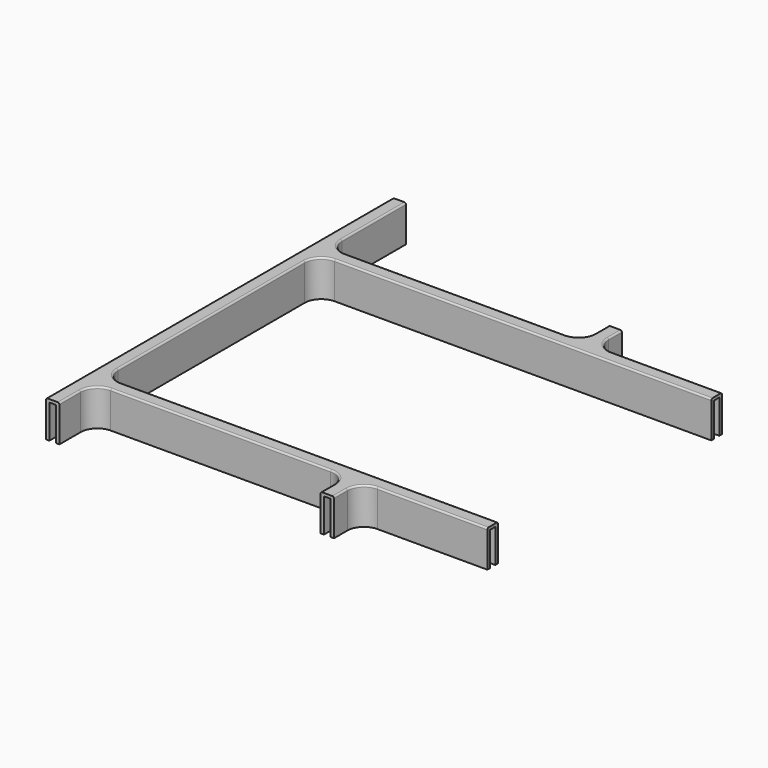
from build123d import *

# Parameters (mm, degrees)
F0_W     = 2
F0_H     = 10
F0_H_2   = 1
F1_DEPTH = 0.9
F0_W_2   = 1
F0_H_3   = 130
F0_W_3   = 76
F0_W_4   = 38
F2_DEPTH = 11
F3_R     = 5
F4_R     = 0.5


with BuildPart() as f1:
    # F0 (on Top) → F1 (new body)
    with BuildSketch(Plane.XY):
        Polygon((-1, -65), (1, -65), (1, -51), (1, -49), (1, 33), (1, 35), (1, 65), (-1, 65), align=None)
        Polygon((1, 35), (1, 33), (2, 33), (79, 33), (81, 33), (120, 33), (120, 35), (82, 35), (81, 35), (79, 35), (78, 35), (2, 35), align=None)
        with Locations((80, 41)):
            Rectangle(F0_W, F0_H)
        with Locations((80, 35.5)):
            Rectangle(F0_W, F0_H_2)
        Polygon((1, -49), (1, -51), (2, -51), (78, -51), (79, -51), (81, -51), (82, -51), (120, -51), (120, -49), (81, -49), (79, -49), (2, -49), align=None)
        with Locations((80, -57)):
            Rectangle(F0_W, F0_H)
        with Locations((80, -51.5)):
            Rectangle(F0_W, F0_H_2)
    extrude(amount=-F1_DEPTH)

    # F0 (on Top) → F2 (join)
    with BuildSketch(Plane.XY):
        Polygon((1, -51), (1, -65), (2, -65), (2, -52), (2, -51), align=None)
        with Locations((-1.5, 0)):
            Rectangle(F0_W_2, F0_H_3)
        Polygon((1, 33), (1, -49), (2, -49), (2, -48), (2, 32), (2, 33), align=None)
        with Locations((40, -51.5)):
            Rectangle(F0_W_3, F0_H_2)
        Polygon((2, 65), (1, 65), (1, 35), (2, 35), (2, 36), align=None)
        Polygon((2, -48), (2, -49), (79, -49), (79, -48), (78, -48), align=None)
        with Locations((78.5, -51.5)):
            Rectangle(F0_W_2, F0_H_2)
        with Locations((78.5, -57)):
            Rectangle(F0_W_2, F0_H)
        Polygon((79, 33), (2, 33), (2, 32), (78, 32), (79, 32), align=None)
        with Locations((80, -48.5)):
            Rectangle(F0_W, F0_H_2)
        with Locations((40, 35.5)):
            Rectangle(F0_W_3, F0_H_2)
        with Locations((80, 32.5)):
            Rectangle(F0_W, F0_H_2)
        Polygon((81, -48), (81, -49), (120, -49), (120, -48), (82, -48), align=None)
        with Locations((81.5, -51.5)):
            Rectangle(F0_W_2, F0_H_2)
        with Locations((81.5, -57)):
            Rectangle(F0_W_2, F0_H)
        with Locations((78.5, 35.5)):
            Rectangle(F0_W_2, F0_H_2)
        with Locations((78.5, 41)):
            Rectangle(F0_W_2, F0_H)
        Polygon((120, 33), (81, 33), (81, 32), (82, 32), (120, 32), align=None)
        with Locations((101, -51.5)):
            Rectangle(F0_W_4, F0_H_2)
        with Locations((81.5, 35.5)):
            Rectangle(F0_W_2, F0_H_2)
        with Locations((81.5, 41)):
            Rectangle(F0_W_2, F0_H)
        with Locations((101, 35.5)):
            Rectangle(F0_W_4, F0_H_2)
    extrude(amount=-F2_DEPTH)

    # F3
    f3_edges = [f1.edges().sort_by_distance(p)[0] for p in [
        (78, -52, -5.5),
        (81, -51, -5.95),
        (82, -52, -5.5),
        (79, -51, -5.95),
        (1, -49, -5.95),
        (1, -51, -5.95),
        (2, -52, -5.5),
        (2, -48, -5.5),
        (2, 36, -5.5),
        (1, 33, -5.95),
        (1, 35, -5.95),
        (2, 32, -5.5),
        (81, 35, -5.95),
        (79, 35, -5.95),
        (82, 36, -5.5),
        (78, 36, -5.5),
    ]]
    fillet(f3_edges, radius=F3_R)

    # F4
    f4_edges = [f1.edges().sort_by_distance(p)[0] for p in [
        (63.5, 32, 0),
        (103.5, 36, 0),
        (82, 43.5, 0),
        (78, 43.5, 0),
        (40, 36, 0),
        (2, 53, 0),
        (40, -52, 0),
        (103.5, -52, 0),
        (-2, 0, 0),
        (2, -61, 0),
        (3.464466, -53.464466, 0),
        (76.535534, -53.464466, 0),
        (78, -59.5, 0),
        (3.464466, 37.464466, 0),
        (82, -59.5, 0),
        (83.464466, -53.464466, 0),
        (76.535534, 37.464466, 0),
        (63.5, -48, 0),
        (3.464466, -46.535534, 0),
        (83.464466, 37.464466, 0),
        (2, -8, 0),
        (3.464466, 30.535534, 0),
    ]]
    fillet(f4_edges, radius=F4_R)


solid = f1.part
